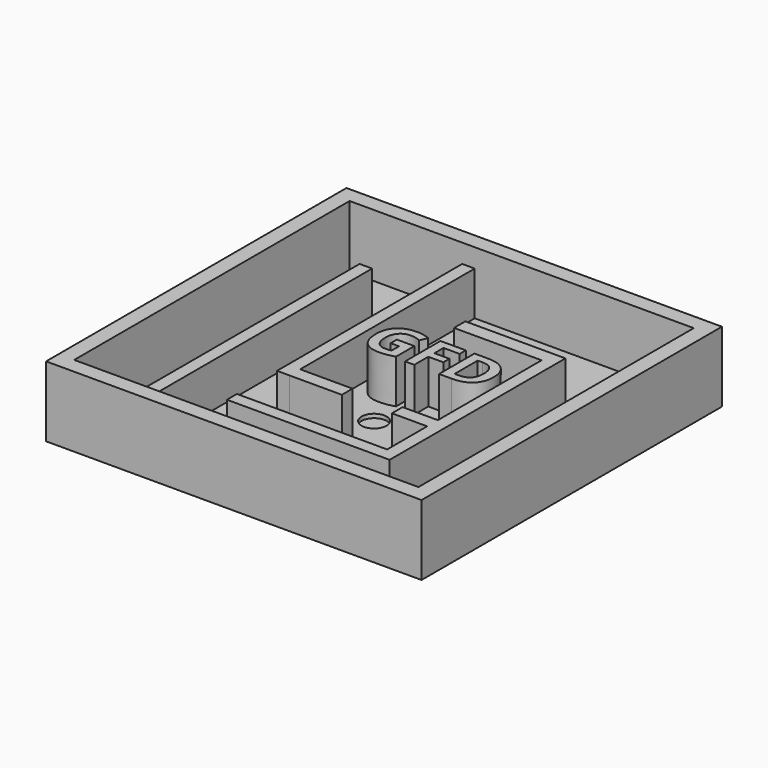
from build123d import *

# Parameters (mm, degrees)
F0_W         = 38.1
F0_H         = 38.1
F1_DEPTH     = 0.79375
F2_W         = 38.1
F2_H         = 38.1
F2_W_2       = 34.925
F2_H_2       = 34.925
F3_DEPTH     = 6.35
F4_W         = 1.27
F4_H         = 29.845
F5_DEPTH     = 4.445
F4_R         = 1.27
F6_DEPTH     = 0.396875
F7_TEXT_SIZE = 6.2871287129
F8_DEPTH     = 4.445


# Not quite as in the source:
# - Text() gives the source's letters only with a copy of the font that has no kerning and outlines rounded to 1/6400 em; it was checked with that copy


with BuildPart() as f1:
    # F0 (on Top) → F1 (new body)
    with BuildSketch(Plane.XY):
        with Locations((8.1274639815, -13.0818684463)):
            Rectangle(F0_W, F0_H)
    extrude(amount=F1_DEPTH)

    # F2 (on face) → F3 (join)
    with BuildSketch(Plane.XY.offset(0.79375)):
        with Locations((8.1274639815, -13.0818684463)):
            Rectangle(F2_W, F2_H)
        with Locations((8.1274639815, -13.0818684463)):
            Rectangle(F2_W_2, F2_H_2, mode=Mode.SUBTRACT)
    extrude(amount=F3_DEPTH)

    # F4 (on face) → F5 (join)
    with BuildSketch(Plane.XY.offset(0.79375)):
        with Locations((-3.6200360185, -15.6218684463)):
            Rectangle(F4_W, F4_H)
        Polygon((3.3649639815, 4.3806315537), (2.0949639815, 4.3806315537), (2.0949639815, -19.1024708379), (3.3649639815, -19.1143684463), (8.6780171841, -19.1143684463), (8.6780171841, -17.7608399319), (3.3649639815, -17.7608399319), align=None)
    extrude(amount=F5_DEPTH)

    # F4 (on face) → F6 (cut)
    with BuildSketch(Plane.XY.offset(0.79375)):
        with Locations((8.1614798129, -14.3776361773)):
            Circle(F4_R)
        with Locations((-6.7950360185, -27.3715220392)):
            Circle(F4_R)
    extrude(amount=-F6_DEPTH, mode=Mode.SUBTRACT)

    # F4 (on face) + F7 (on face) → F8 (join)
    with BuildSketch(Plane.XY.offset(0.79375)):
        Polygon((2.0949639815, -24.1943684463), (2.0949639815, -25.4643684463), (3.3649639815, -25.4643684463), (18.6049639815, -25.4643684463), (18.6049639815, -24.1943684463), (18.6049639815, -3.1644518204), (17.3349639815, -3.1644518204), (8.4449639815, -3.1644518204), (8.4449639815, -4.6015088492), (17.3349639815, -4.6015088492), (17.3349639815, -17.7608399319), (13.7580171841, -17.7608399319), (13.7580171841, -19.1143684463), (17.3349639815, -19.1143684463), (17.3349639815, -22.3487187177), (17.3349639815, -24.1943684463), (3.3649639815, -24.1943684463), align=None)
    with BuildSketch(Plane.XY.offset(0.79375)):
        with Locations((3.8913410906, -11.5124595571)):
            Text('GFD', F7_TEXT_SIZE, font='Open Sans', font_style=FontStyle.BOLD, text_align=(TextAlign.LEFT, TextAlign.BOTTOM))
    extrude(amount=F8_DEPTH)


solid = f1.part
